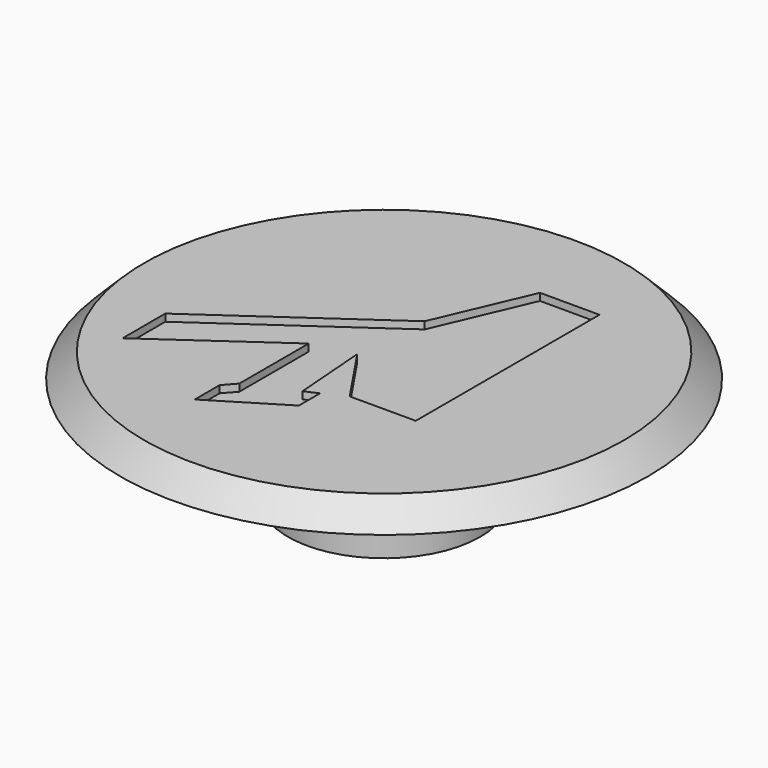
from build123d import *

# Parameters (mm, degrees)
F0_R     = 4
F1_DEPTH = 3.5
F2_R     = 6
F3_DEPTH = 1
F4_R     = 11
F5_DEPTH = 1
F6_SIZE  = 0.99999
F8_DEPTH = 0.3


# Not quite as in the source:
# - a fillet or chamfer is up to 0.001 mm smaller than in the source, because OpenCascade refuses the exact size


with BuildPart() as f1:
    # F0 (on Top) → F1 (new body)
    with BuildSketch(Plane.XY):
        Circle(F0_R)
    extrude(amount=F1_DEPTH)

    # F2 (on face) → F3 (join)
    with BuildSketch(Plane.XY.offset(3.5)):
        Circle(F2_R)
    extrude(amount=F3_DEPTH)

    # F4 (on face) → F5 (join)
    with BuildSketch(Plane.XY.offset(4.5)):
        Circle(F4_R)
    extrude(amount=F5_DEPTH)

    # F6 (size 1 in the source; OpenCascade refuses exactly that, so slightly less here)
    f6_edges = [f1.edges().sort_by_distance(p)[0] for p in [
        (-11, 0, 5.5),
    ]]
    chamfer(f6_edges, length=F6_SIZE)

    # F7 (on face) → F8 (cut)
    with BuildSketch(Plane.XY.offset(5.5)):
        Polygon((1.3699667839, 6.4073562332), (-0.3065554774, 2.496608533), (-7.2352840317, -2.3525079081), (-7.2352840317, -4.5790599288), (-2.2722620734, -1.0865629438), (-2.2722620734, -4.7009375549), (-2.7038290382, -5.1864506813), (-2.7038290382, -6.4811520415), (0.2092490221, -4.7009375549), (0.2092490221, -3.5950467127), (-0.3302100332, -3.8378033924), (-0.57296648, -0.6819687688), (1.099356149, -3.1634797479), (2.4749761405, -3.1634797479), (3.8502510524, -3.1634797479), (3.8502510524, 4.6872763105), (3.8502510524, 6.4073562332), align=None)
    extrude(amount=-F8_DEPTH, mode=Mode.SUBTRACT)


solid = f1.part
